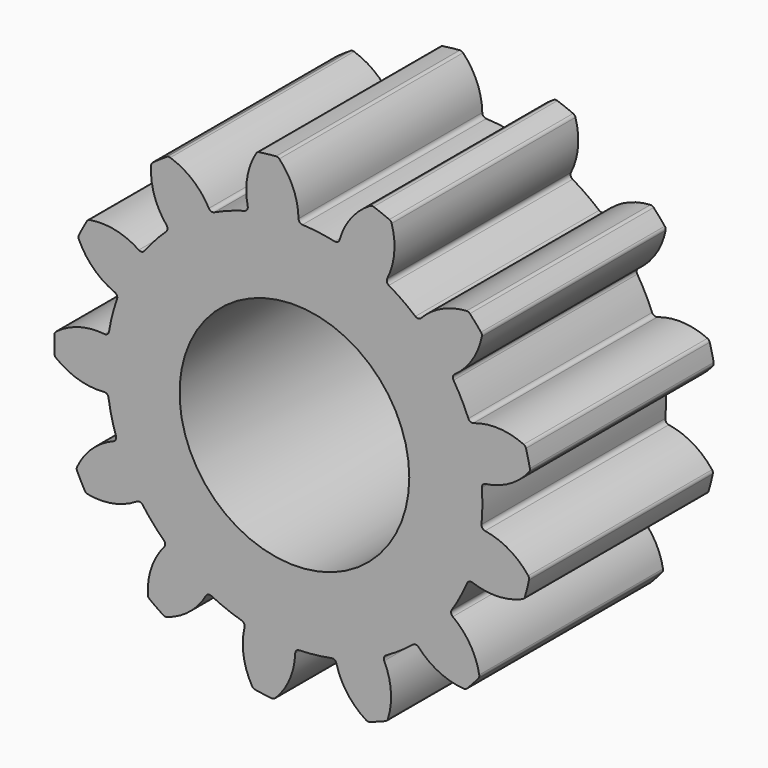
from build123d import *

# Parameters (mm, degrees)
F1_DEPTH = 2.2
F2_R     = 1.1
F3_DEPTH = 2.201


# Not quite as in the source:
# - a feature names something its author has since deleted; it is built from what else it names


with BuildPart() as f1:
    # F0 (on Front) → F1 (new body)
    with BuildSketch(Plane.XZ):
        with BuildLine():
            ThreePointArc((0.039122928, 1.8376830625), (-0.0105540318, 2.0770952736), (-0.1451690317, 2.2812148684))
            ThreePointArc((-0.1451690317, 2.2812148684), (-0.159702791, 2.2907302121), (-0.1768997755, 2.2931869678))
            ThreePointArc((-0.1768997755, 2.2931869678), (-0.257518295, 2.2855380828), (-0.337817577, 2.2750558861))
            ThreePointArc((-0.337817577, 2.2750558861), (-0.3540367176, 2.2688340373), (-0.366088722, 2.2563231974))
            ThreePointArc((-0.366088722, 2.2563231974), (-0.45190776, 2.0273666515), (-0.4470649859, 1.7829028409))
            ThreePointArc((-0.4470649859, 1.7829028409), (-0.4520346154, 1.7537914646), (-0.475624931, 1.7360244598))
            ThreePointArc((-0.475624931, 1.7360244598), (-0.6237394012, 1.688475395), (-0.7671953061, 1.6283154984))
            ThreePointArc((-0.7671953061, 1.6283154984), (-1.0096932785, 1.4901407595), (-1.2279157548, 1.316139392))
            ThreePointArc((-1.2279157548, 1.316139392), (-1.3369674527, 1.2052045596), (-1.4360336502, 1.0852683334))
            ThreePointArc((-1.4360336502, 1.0852683334), (-1.5865419381, 0.8502262514), (-1.6989058772, 0.5947426506))
            ThreePointArc((-1.6989058772, 0.5947426506), (-1.743912373, 0.4458358839), (-1.775893991, 0.2935992722))
            ThreePointArc((-1.775893991, 0.2935992722), (-1.7999329596, 0.0155351554), (-1.7806971371, -0.2629024645))
            ThreePointArc((-1.7806971371, -0.2629024645), (-1.751347985, -0.4156684199), (-1.7089184204, -0.565329844))
            ThreePointArc((-1.7089184204, -0.565329844), (-1.6009810315, -0.8227148575), (-1.4545521427, -1.0603197934))
            ThreePointArc((-1.4545521427, -1.0603197934), (-1.3575708798, -1.181948098), (-1.2504502343, -1.2947487059))
            ThreePointArc((-1.2504502343, -1.2947487059), (-1.0352636431, -1.4724908113), (-0.7951867816, -1.6148306358))
            ThreePointArc((-0.7951867816, -1.6148306358), (-0.6527906465, -1.6774577109), (-0.5055189691, -1.7275562427))
            ThreePointArc((-0.5055189691, -1.7275562427), (-0.2323798303, -1.7849368657), (0.0463462881, -1.7994032404))
            ThreePointArc((0.0463462881, -1.7994032404), (0.201536057, -1.7886819778), (0.3552205997, -1.7646014637))
            ThreePointArc((0.3552205997, -1.7646014637), (0.6237394012, -1.688475395), (0.8772619817, -1.5717542478))
            ThreePointArc((0.8772619817, -1.5717542478), (1.0096932785, -1.4901407595), (1.13458341, -1.397397755))
            ThreePointArc((1.13458341, -1.397397755), (1.3369674527, -1.2052045596), (1.5072075275, -0.9840352987))
            ThreePointArc((1.5072075275, -0.9840352987), (1.5865419381, -0.8502262514), (1.6540268343, -0.7100670611))
            ThreePointArc((1.6540268343, -0.7100670611), (1.743912373, -0.4458358839), (1.7918699925, -0.1708857215))
            ThreePointArc((1.7918699925, -0.1708857215), (1.7999329596, -0.0155351554), (1.7945526441, 0.1399314392))
            ThreePointArc((1.7945526441, 0.1399314392), (1.751347985, 0.4156684199), (1.6660366367, 0.681411715))
            ThreePointArc((1.6660366367, 0.681411715), (1.6009810315, 0.8227148575), (1.5239680698, 0.9578733332))
            ThreePointArc((1.5239680698, 0.9578733332), (1.3575708798, 1.181948098), (1.1585343652, 1.3776059395))
            ThreePointArc((1.1585343652, 1.3776059395), (1.0352636431, 1.4724908113), (0.9042607765, 1.5563779901))
            ThreePointArc((0.9042607765, 1.5563779901), (0.6527906465, 1.6774577109), (0.3856258326, 1.7582072452))
            ThreePointArc((0.3856258326, 1.7582072452), (0.2323798303, 1.7849368657), (0.0773982368, 1.7983352059))
            ThreePointArc((0.0773982368, 1.7983352059), (0.0504458492, 1.8104074157), (0.039122928, 1.8376830625))
        make_face()
        with BuildLine():
            ThreePointArc((-1.2279157548, 1.316139392), (-1.0096932785, 1.4901407595), (-0.7671953061, 1.6283154984))
            ThreePointArc((-0.7671953061, 1.6283154984), (-0.7966706958, 1.6264795102), (-0.8193722697, 1.6453688721))
            ThreePointArc((-0.8193722697, 1.6453688721), (-0.9746194353, 1.8342718227), (-1.1886742036, 1.9524520381))
            ThreePointArc((-1.1886742036, 1.9524520381), (-1.2059652091, 1.9541232819), (-1.222334094, 1.9483067938))
            ThreePointArc((-1.222334094, 1.9483067938), (-1.2901636337, 1.9040687483), (-1.3563937971, 1.8574702871))
            ThreePointArc((-1.3563937971, 1.8574702871), (-1.3678636956, 1.8444237031), (-1.3727211383, 1.8277450588))
            ThreePointArc((-1.3727211383, 1.8277450588), (-1.3423087103, 1.5851320101), (-1.2244126493, 1.3709206053))
            ThreePointArc((-1.2244126493, 1.3709206053), (-1.2152843065, 1.3428342597), (-1.2279157548, 1.316139392))
        make_face()
        with BuildLine():
            ThreePointArc((-1.7806971371, -0.2629024645), (-1.7999329596, 0.0155351554), (-1.775893991, 0.2935992722))
            ThreePointArc((-1.775893991, 0.2935992722), (-1.7911269321, 0.2682985419), (-1.819568536, 0.2603458935))
            ThreePointArc((-1.819568536, 0.2603458935), (-2.0632230584, 0.2398890878), (-2.2820804367, 0.1308594811))
            ThreePointArc((-2.2820804367, 0.1308594811), (-2.293278254, 0.1175786373), (-2.2977899646, 0.1008031673))
            ThreePointArc((-2.2977899646, 0.1008031673), (-2.2999143372, 0.0198504764), (-2.2991875764, -0.0611268226))
            ThreePointArc((-2.2991875764, -0.0611268226), (-2.2949660933, -0.0779776684), (-2.2839991801, -0.0914498153))
            ThreePointArc((-2.2839991801, -0.0914498153), (-2.0670563272, -0.2042407978), (-1.8237912011, -0.2289001891))
            ThreePointArc((-1.8237912011, -0.2289001891), (-1.7954911021, -0.2373425731), (-1.7806971371, -0.2629024645))
        make_face()
        with BuildLine():
            ThreePointArc((-0.7951867816, -1.6148306358), (-1.0352636431, -1.4724908113), (-1.2504502343, -1.2947487059))
            ThreePointArc((-1.2504502343, -1.2947487059), (-1.2382814383, -1.3216576237), (-1.2478932095, -1.349582224))
            ThreePointArc((-1.2478932095, -1.349582224), (-1.369469133, -1.5617267549), (-1.404064687, -1.8037787221))
            ThreePointArc((-1.404064687, -1.8037787221), (-1.399495852, -1.8205387242), (-1.3882528546, -1.8337813424))
            ThreePointArc((-1.3882528546, -1.8337813424), (-1.3228368773, -1.8815160366), (-1.2557810195, -1.9269182731))
            ThreePointArc((-1.2557810195, -1.9269182731), (-1.2395149695, -1.933016432), (-1.2221976933, -1.9316438911))
            ThreePointArc((-1.2221976933, -1.9316438911), (-1.0061349477, -1.8171760042), (-0.8476503242, -1.6309808612))
            ThreePointArc((-0.8476503242, -1.6309808612), (-0.8246260898, -1.612486157), (-0.7951867816, -1.6148306358))
        make_face()
        with BuildLine():
            ThreePointArc((0.0073975122, -1.8380845787), (0.0191895417, -1.8110084362), (0.0463462881, -1.7994032404))
            ThreePointArc((0.0463462881, -1.7994032404), (-0.2323798303, -1.7849368657), (-0.5055189691, -1.7275562427))
            ThreePointArc((-0.5055189691, -1.7275562427), (-0.4822388378, -1.7457277846), (-0.4777724297, -1.774920603))
            ThreePointArc((-0.4777724297, -1.774920603), (-0.4868340843, -2.019264405), (-0.4049797681, -2.2496681335))
            ThreePointArc((-0.4049797681, -2.2496681335), (-0.3931455043, -2.2623851349), (-0.377036173, -2.2688860095))
            ThreePointArc((-0.377036173, -2.2688860095), (-0.2969297831, -2.2807526617), (-0.2164552985, -2.2897919346))
            ThreePointArc((-0.2164552985, -2.2897919346), (-0.1992184707, -2.2876323759), (-0.1845226357, -2.2783693117))
            ThreePointArc((-0.1845226357, -2.2783693117), (-0.0464044552, -2.076603667), (0.0073975122, -1.8380845787))
        make_face()
        with BuildLine():
            ThreePointArc((0.8607506676, -1.6241052705), (0.8586090804, -1.5946505077), (0.8772619817, -1.5717542478))
            ThreePointArc((0.8772619817, -1.5717542478), (0.6237394012, -1.688475395), (0.3552205997, -1.7646014637))
            ThreePointArc((0.3552205997, -1.7646014637), (0.3842788689, -1.7698727484), (0.401800256, -1.793646062))
            ThreePointArc((0.401800256, -1.793646062), (0.5073287861, -2.0142129148), (0.6868811351, -2.180185687))
            ThreePointArc((0.6868811351, -2.180185687), (0.7032697406, -2.1859463759), (0.7205549521, -2.1842162349))
            ThreePointArc((0.7205549521, -2.1842162349), (0.7970003459, -2.157496338), (0.8724577228, -2.1281018589))
            ThreePointArc((0.8724577228, -2.1281018589), (0.8867165788, -2.1181793113), (0.8954243339, -2.1031477803))
            ThreePointArc((0.8954243339, -2.1031477803), (0.9239567387, -1.8603064554), (0.8607506676, -1.6241052705))
        make_face()
        with BuildLine():
            ThreePointArc((1.5169162183, -1.0380630175), (1.5013316261, -1.0129773655), (1.5072075275, -0.9840352987))
            ThreePointArc((1.5072075275, -0.9840352987), (1.3369674527, -1.2052045596), (1.13458341, -1.397397755))
            ThreePointArc((1.13458341, -1.397397755), (1.1627629177, -1.3885611948), (1.1893253453, -1.401468824))
            ThreePointArc((1.1893253453, -1.401468824), (1.3852687455, -1.5477295196), (1.6213858481, -1.6112489736))
            ThreePointArc((1.6213858481, -1.6112489736), (1.6385743632, -1.6087336456), (1.6530756213, -1.5991688436))
            ThreePointArc((1.6530756213, -1.5991688436), (1.7083473006, -1.5399836039), (1.7615011941, -1.4788892938))
            ThreePointArc((1.7615011941, -1.4788892938), (1.7695155463, -1.4634768934), (1.7702403797, -1.4461204381))
            ThreePointArc((1.7702403797, -1.4461204381), (1.6826505787, -1.2178354541), (1.5169162183, -1.0380630175))
        make_face()
        with BuildLine():
            ThreePointArc((1.8255745442, -0.2142130372), (1.8001171894, -0.1992433165), (1.7918699925, -0.1708857215))
            ThreePointArc((1.7918699925, -0.1708857215), (1.743912373, -0.4458358839), (1.6540268343, -0.7100670611))
            ThreePointArc((1.6540268343, -0.7100670611), (1.6748719949, -0.6891470055), (1.7043903309, -0.6882319679))
            ThreePointArc((1.7043903309, -0.6882319679), (1.9458603297, -0.7266799437), (2.1844506031, -0.6731945381))
            ThreePointArc((2.1844506031, -0.6731945381), (2.1985013461, -0.6629794245), (2.2068965874, -0.6477711422))
            ThreePointArc((2.2068965874, -0.6477711422), (2.2283324766, -0.569679185), (2.2470059702, -0.4908810139))
            ThreePointArc((2.2470059702, -0.4908810139), (2.2469398271, -0.473509556), (2.2395156882, -0.4578043312))
            ThreePointArc((2.2395156882, -0.4578043312), (2.0558694492, -0.2963730267), (1.8255745442, -0.2142130372))
        make_face()
        with BuildLine():
            ThreePointArc((1.7160157425, 0.6587105685), (1.6865175983, 0.6601349751), (1.6660366367, 0.681411715))
            ThreePointArc((1.6660366367, 0.681411715), (1.751347985, 0.4156684199), (1.7945526441, 0.1399314392))
            ThreePointArc((1.7945526441, 0.1399314392), (1.8032880825, 0.1681424577), (1.8290000318, 0.1826705379))
            ThreePointArc((1.8290000318, 0.1826705379), (2.0606787625, 0.2608432499), (2.2470840504, 0.4190806532))
            ThreePointArc((2.2470840504, 0.4190806532), (2.2547781655, 0.434655393), (2.2551441412, 0.4520231213))
            ThreePointArc((2.2551441412, 0.4520231213), (2.2378335365, 0.5311318698), (2.2177487579, 0.6095821904))
            ThreePointArc((2.2177487579, 0.6095821904), (2.209617272, 0.6249331143), (2.1957449416, 0.6353892309))
            ThreePointArc((2.1957449416, 0.6353892309), (1.9581134048, 0.6929848894), (1.7160157425, 0.6587105685))
        make_face()
        with BuildLine():
            ThreePointArc((1.2133384145, 1.3807315211), (1.1865571502, 1.3682842994), (1.1585343652, 1.3776059395))
            ThreePointArc((1.1585343652, 1.3776059395), (1.3575708798, 1.181948098), (1.5239680698, 0.9578733332))
            ThreePointArc((1.5239680698, 0.9578733332), (1.5185926024, 0.9869125101), (1.5346078672, 1.0117254249))
            ThreePointArc((1.5346078672, 1.0117254249), (1.7034205247, 1.1886103985), (1.794937622, 1.4153495174))
            ThreePointArc((1.794937622, 1.4153495174), (1.7945124802, 1.4327158981), (1.7867653498, 1.4482643352))
            ThreePointArc((1.7867653498, 1.4482643352), (1.7346739019, 1.5102670141), (1.6804320319, 1.5703974612))
            ThreePointArc((1.6804320319, 1.5703974612), (1.6660980287, 1.5802111393), (1.6489554905, 1.5830227774))
            ThreePointArc((1.6489554905, 1.5830227774), (1.4117771772, 1.5235883187), (1.2133384145, 1.3807315211))
        make_face()
        with BuildLine():
            ThreePointArc((0.432699878, 1.786443522), (0.4147707585, 1.7629761804), (0.3856258326, 1.7582072452))
            ThreePointArc((0.3856258326, 1.7582072452), (0.6527906465, 1.6774577109), (0.9042607765, 1.5563779901))
            ThreePointArc((0.9042607765, 1.5563779901), (0.886005858, 1.5795928001), (0.8886555343, 1.6090062097))
            ThreePointArc((0.8886555343, 1.6090062097), (0.9559291731, 1.844081229), (0.9315926158, 2.0873788639))
            ThreePointArc((0.9315926158, 2.0873788639), (0.9231456119, 2.1025584571), (0.9090601496, 2.1127256434))
            ThreePointArc((0.9090601496, 2.1127256434), (0.8341213816, 2.1434181862), (0.7581485788, 2.171453599))
            ThreePointArc((0.7581485788, 2.171453599), (0.7408958057, 2.173481836), (0.7244102086, 2.1680048831))
            ThreePointArc((0.7244102086, 2.1680048831), (0.5420198121, 2.0051560255), (0.432699878, 1.786443522))
        make_face()
        with BuildLine():
            ThreePointArc((-1.6989058772, 0.5947426506), (-1.5865419381, 0.8502262514), (-1.4360336502, 1.0852683334))
            ThreePointArc((-1.4360336502, 1.0852683334), (-1.4612795853, 1.0699447501), (-1.4901591549, 1.076120502))
            ThreePointArc((-1.4901591549, 1.076120502), (-1.7154112715, 1.1712388026), (-1.9598684406, 1.1764059755))
            ThreePointArc((-1.9598684406, 1.1764059755), (-1.9759555312, 1.1698502574), (-1.9877464022, 1.1570930129))
            ThreePointArc((-1.9877464022, 1.1570930129), (-2.027248032, 1.0864002101), (-2.0642365445, 1.0143606302))
            ThreePointArc((-2.0642365445, 1.0143606302), (-2.0683295854, 0.9974781262), (-2.0648796848, 0.9804525539))
            ThreePointArc((-2.0648796848, 0.9804525539), (-1.9252029116, 0.7797627281), (-1.7212621305, 0.6448769804))
            ThreePointArc((-1.7212621305, 0.6448769804), (-1.7001270088, 0.6242499088), (-1.6989058772, 0.5947426506))
        make_face()
        with BuildLine():
            ThreePointArc((-1.4545521427, -1.0603197934), (-1.6009810315, -0.8227148575), (-1.7089184204, -0.565329844))
            ThreePointArc((-1.7089184204, -0.565329844), (-1.7106486842, -0.5948116288), (-1.7321366938, -0.6150708217))
            ThreePointArc((-1.7321366938, -0.6150708217), (-1.9383753071, -0.7464163261), (-2.0814953069, -0.9446653433))
            ThreePointArc((-2.0814953069, -0.9446653433), (-2.0852385658, -0.9616288317), (-2.0814375375, -0.9785794691))
            ThreePointArc((-2.0814375375, -0.9785794691), (-2.0456979847, -1.0512467623), (-2.0074224428, -1.122610857))
            ThreePointArc((-2.0074224428, -1.122610857), (-1.9958535266, -1.135569719), (-1.9798819884, -1.1424021339))
            ThreePointArc((-1.9798819884, -1.1424021339), (-1.7353720489, -1.1414552182), (-1.5085116865, -1.0502390838))
            ThreePointArc((-1.5085116865, -1.0502390838), (-1.4795298219, -1.0445627318), (-1.4545521427, -1.0603197934))
        make_face()
    extrude(amount=F1_DEPTH)

    # F2 (on face) → F3 (cut, through all)
    with BuildSketch(Plane.XZ.offset(2.2)):
        Circle(F2_R)
    extrude(amount=-F3_DEPTH, mode=Mode.SUBTRACT)


solid = f1.part
